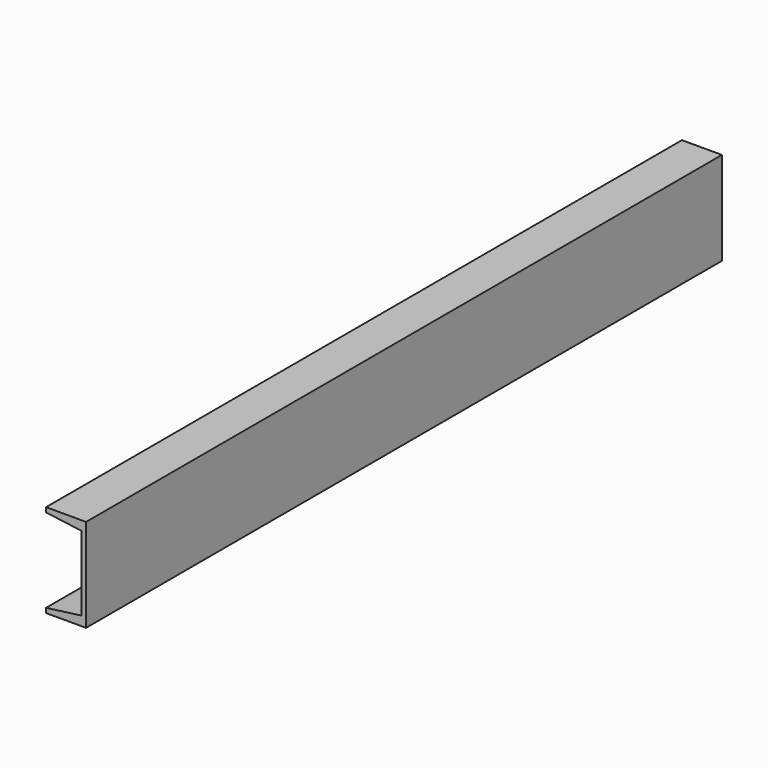
from build123d import *

# Parameters (mm, degrees)
F1_DEPTH = 596.5
F2_SIZE2 = 52.99999
F2_SIZE  = 6.99999
F3_SIZE2 = 6.99999
F3_SIZE  = 52.99999


# Not quite as in the source:
# - a fillet or chamfer is up to 0.001 mm smaller than in the source, because OpenCascade refuses the exact size


with BuildPart() as f1:
    # F0 (on Front) → F1 (new body, symmetric)
    with BuildSketch(Plane.XZ):
        Polygon((-60, 0), (0, 0), (0, 140), (-60, 140), (-60, 126), (-7, 126), (-7, 14), (-60, 14), align=None)
    extrude(amount=F1_DEPTH, both=True)

    # F2 (size 7 and 53 in the source; OpenCascade refuses exactly that, so slightly less here)
    f2_edges = [f1.edges().sort_by_distance(p)[0] for p in [
        (-60, 0, 14),
    ]]
    f2_side = f1.faces().sort_by_distance((-60, 0, 7))[0]
    chamfer(f2_edges, length=F2_SIZE, length2=F2_SIZE2, reference=f2_side)

    # F3 (size 53 and 7 in the source; OpenCascade refuses exactly that, so slightly less here)
    f3_edges = [f1.edges().sort_by_distance(p)[0] for p in [
        (-60, 0, 126),
    ]]
    f3_side = f1.faces().sort_by_distance((-33.5, 0, 126))[0]
    chamfer(f3_edges, length=F3_SIZE, length2=F3_SIZE2, reference=f3_side)


solid = f1.part
